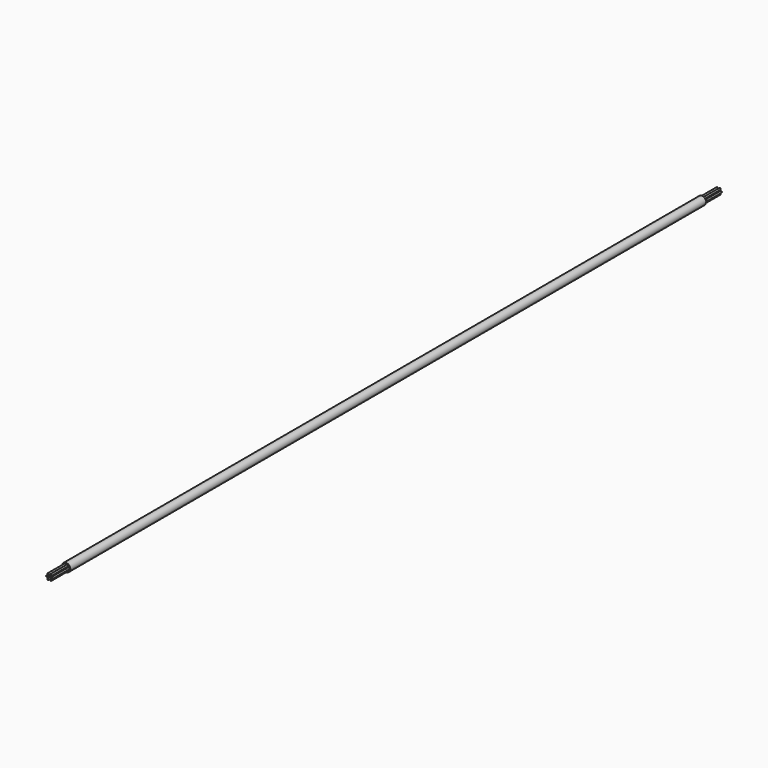
from build123d import *

# Parameters (mm, degrees)
F0_R     = 1.6
F0_R_2   = 0.32131
F1_DEPTH = 305
F2_R     = 0.32131
F3_DEPTH = 8
F4_R     = 0.32131
F5_DEPTH = 8


with BuildPart() as f1:
    # F0 (on Front) → F1 (new body)
    with BuildSketch(Plane.XZ):
        Circle(F0_R)
        with Locations((-0.481965, -0.8347878675)):
            Circle(F0_R_2, mode=Mode.SUBTRACT)
        with Locations((0.481965, -0.8347878675)):
            Circle(F0_R_2, mode=Mode.SUBTRACT)
        with Locations((-0.96393, 0)):
            Circle(F0_R_2, mode=Mode.SUBTRACT)
        with Locations((-0.481965, 0.8347878675)):
            Circle(F0_R_2, mode=Mode.SUBTRACT)
        with Locations((0.96393, 0)):
            Circle(F0_R_2, mode=Mode.SUBTRACT)
        with Locations((0.481965, 0.8347878675)):
            Circle(F0_R_2, mode=Mode.SUBTRACT)
    extrude(amount=F1_DEPTH)


with BuildPart() as f3:
    # F2 (on face) → F3 (new body)
    with BuildSketch(Plane.XZ.offset(305)):
        with Locations((-0.481965, 0.8347878675)):
            Circle(F2_R)
    extrude(amount=F3_DEPTH)


with BuildPart() as f3b:
    # F2 (on face) → F3, piece 2 (new body)
    with BuildSketch(Plane.XZ.offset(305)):
        with Locations((0.481965, 0.8347878675)):
            Circle(F2_R)
    extrude(amount=F3_DEPTH)


with BuildPart() as f3c:
    # F2 (on face) → F3, piece 3 (new body)
    with BuildSketch(Plane.XZ.offset(305)):
        with Locations((-0.96393, 0)):
            Circle(F2_R)
    extrude(amount=F3_DEPTH)


with BuildPart() as f3d:
    # F2 (on face) → F3, piece 4 (new body)
    with BuildSketch(Plane.XZ.offset(305)):
        with Locations((-0.481965, -0.8347878675)):
            Circle(F2_R)
    extrude(amount=F3_DEPTH)


with BuildPart() as f3e:
    # F2 (on face) → F3, piece 5 (new body)
    with BuildSketch(Plane.XZ.offset(305)):
        with Locations((0.481965, -0.8347878675)):
            Circle(F2_R)
    extrude(amount=F3_DEPTH)


with BuildPart() as f3f:
    # F2 (on face) → F3, piece 6 (new body)
    with BuildSketch(Plane.XZ.offset(305)):
        with Locations((0.96393, 0)):
            Circle(F2_R)
    extrude(amount=F3_DEPTH)


with BuildPart() as f5:
    # F4 (on face) → F5 (new body)
    with BuildSketch(Plane(origin=(0, 0, 0), x_dir=(-1, 0, 0), z_dir=(0, 1, 0))):
        with Locations((0.481965, -0.8347878675)):
            Circle(F4_R)
    extrude(amount=F5_DEPTH)


with BuildPart() as f5b:
    # F4 (on face) → F5, piece 2 (new body)
    with BuildSketch(Plane(origin=(0, 0, 0), x_dir=(-1, 0, 0), z_dir=(0, 1, 0))):
        with Locations((-0.481965, -0.8347878675)):
            Circle(F4_R)
    extrude(amount=F5_DEPTH)


with BuildPart() as f5c:
    # F4 (on face) → F5, piece 3 (new body)
    with BuildSketch(Plane(origin=(0, 0, 0), x_dir=(-1, 0, 0), z_dir=(0, 1, 0))):
        with Locations((0.96393, 0)):
            Circle(F4_R)
    extrude(amount=F5_DEPTH)


with BuildPart() as f5d:
    # F4 (on face) → F5, piece 4 (new body)
    with BuildSketch(Plane(origin=(0, 0, 0), x_dir=(-1, 0, 0), z_dir=(0, 1, 0))):
        with Locations((0.481965, 0.8347878675)):
            Circle(F4_R)
    extrude(amount=F5_DEPTH)


with BuildPart() as f5e:
    # F4 (on face) → F5, piece 5 (new body)
    with BuildSketch(Plane(origin=(0, 0, 0), x_dir=(-1, 0, 0), z_dir=(0, 1, 0))):
        with Locations((-0.96393, 0)):
            Circle(F4_R)
    extrude(amount=F5_DEPTH)


with BuildPart() as f5f:
    # F4 (on face) → F5, piece 6 (new body)
    with BuildSketch(Plane(origin=(0, 0, 0), x_dir=(-1, 0, 0), z_dir=(0, 1, 0))):
        with Locations((-0.481965, 0.8347878675)):
            Circle(F4_R)
    extrude(amount=F5_DEPTH)


solid = Compound([f1.part, f3.part, f3b.part, f3c.part, f3d.part, f3e.part, f3f.part, f5.part, f5b.part, f5c.part, f5d.part, f5e.part, f5f.part])
